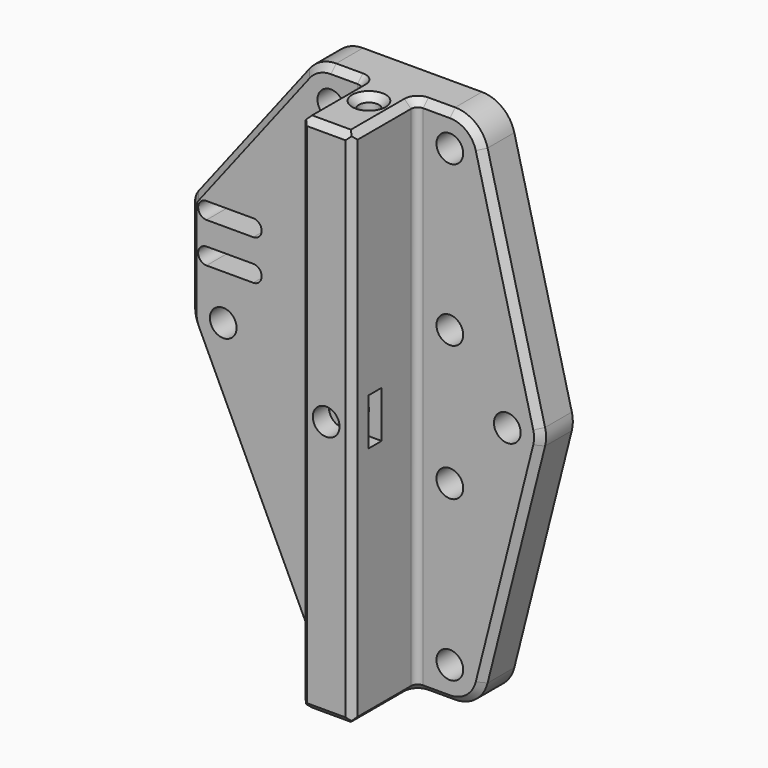
from build123d import *

# Parameters (mm, degrees)
F0_R          = 2
F1_DEPTH      = 6
F2_W          = 7.8
F2_H          = 78
F3_DEPTH      = 12
F4_R          = 2
F5_DEPTH      = 12
F6_W          = 2.5
F6_H          = 7
F7_DEPTH      = 33.901
F8_R          = 1.5
F9_DEPTH      = 39.001
F9_DEPTH_BACK = 39.001
F10_DEPTH     = 2.5
F11_SIZE      = 1
F12_R         = 1
F13_SIZE      = 1
F14_SIZE      = 1
F15_W         = 13.75
F15_H         = 4
F16_DEPTH     = 2


# Not quite as in the source:
# - a feature names something its author has since deleted; it is built from what else it names


with BuildPart() as f1:
    # F0 (on Front) → F1 (new body)
    with BuildSketch(Plane.XZ):
        with BuildLine():
            Line((22.3473393815, 1.2260917259), (13.7473393815, 35.2260917259))
            ThreePointArc((13.7473393815, 35.2260917259), (11.9716071828, 37.9452793709), (8.9, 39))
            Line((8.9, 39), (-8.9, 39))
            ThreePointArc((-8.9, 39), (-11.1047505583, 38.4876580725), (-12.8576666563, 37.0556299903))
            Line((-12.8576666563, 37.0556299903), (-29.4788333281, 15.5278149952))
            ThreePointArc((-29.4788333281, 15.5278149952), (-29.8661237626, 14.8071296921), (-30, 14))
            Line((-30, 14), (-30, 0))
            ThreePointArc((-30, 0), (-29.8782578321, -1.0966314436), (-29.5189597908, -2.1398603715))
            Line((-29.5189597908, -2.1398603715), (-13.4189597908, -36.1398603715))
            ThreePointArc((-13.4189597908, -36.1398603715), (-11.5740136632, -38.2248847237), (-8.9, -39))
            Line((-8.9, -39), (8.9, -39))
            ThreePointArc((8.9, -39), (11.9716071828, -37.9452793709), (13.7473393815, -35.2260917259))
            Line((13.7473393815, -35.2260917259), (22.3473393815, -1.2260917259))
            ThreePointArc((22.3473393815, -1.2260917259), (22.5, 0), (22.3473393815, 1.2260917259))
        make_face()
        with Locations((-8.9, -34)):
            Circle(F0_R, mode=Mode.SUBTRACT)
        with Locations((-8.9, -10.1)):
            Circle(F0_R, mode=Mode.SUBTRACT)
        with Locations((8.9, -34)):
            Circle(F0_R, mode=Mode.SUBTRACT)
        with Locations((8.9, -10.1)):
            Circle(F0_R, mode=Mode.SUBTRACT)
        with Locations((-25, 0)):
            Circle(F0_R, mode=Mode.SUBTRACT)
        with BuildLine():
            ThreePointArc((-20.5, 9.25), (-19.25, 8), (-20.5, 6.75))
            Line((-20.5, 6.75), (-27.5, 6.75))
            ThreePointArc((-27.5, 6.75), (-28.75, 8), (-27.5, 9.25))
            Line((-27.5, 9.25), (-20.5, 9.25))
        make_face(mode=Mode.SUBTRACT)
        with BuildLine():
            ThreePointArc((-27.5, 12.75), (-28.75, 14), (-27.5, 15.25))
            Line((-27.5, 15.25), (-20.5, 15.25))
            ThreePointArc((-20.5, 15.25), (-19.25, 14), (-20.5, 12.75))
            Line((-20.5, 12.75), (-27.5, 12.75))
        make_face(mode=Mode.SUBTRACT)
        with Locations((-8.9, 10.1)):
            Circle(F0_R, mode=Mode.SUBTRACT)
        with Locations((-8.9, 34)):
            Circle(F0_R, mode=Mode.SUBTRACT)
        with Locations((8.9, 10.1)):
            Circle(F0_R, mode=Mode.SUBTRACT)
        with Locations((17.5, 0)):
            Circle(F0_R, mode=Mode.SUBTRACT)
        with Locations((8.9, 34)):
            Circle(F0_R, mode=Mode.SUBTRACT)
    extrude(amount=F1_DEPTH)

    # F2 (on face) → F3 (join)
    with BuildSketch(Plane.XZ.offset(6)):
        Rectangle(F2_W, F2_H)
    extrude(amount=F3_DEPTH)

    # F4 (on face) → F5 (cut, through all)
    with BuildSketch(Plane.XZ.offset(18)):
        Circle(F4_R)
    extrude(amount=-F5_DEPTH, mode=Mode.SUBTRACT)

    # F6 (on face) → F7 (cut, through all)
    with BuildSketch(Plane.YZ.offset(3.9)):
        with Locations((-13.75, 0)):
            Rectangle(F6_W, F6_H)
    extrude(amount=-F7_DEPTH, mode=Mode.SUBTRACT)

    # F8 (on Top) → F9 (cut, two sides)
    with BuildSketch(Plane.XY) as f9_sk:
        with Locations((0, -10)):
            Circle(F8_R)
    extrude(amount=-F9_DEPTH, mode=Mode.SUBTRACT)
    extrude(f9_sk.sketch, amount=F9_DEPTH_BACK, mode=Mode.SUBTRACT)

    # F10 (add): a face of the model
    f10_faces = [f1.faces().sort_by_distance(p)[0] for p in [
        (0, -6, 0),
    ]]
    extrude(f10_faces, amount=F10_DEPTH)

    # F11
    f11_edges = [f1.edges().sort_by_distance(p)[0] for p in [
        (3.9, -18, 0),
        (-3.9, -18, 0),
    ]]
    chamfer(f11_edges, length=F11_SIZE)

    # F12
    f12_edges = [f1.edges().sort_by_distance(p)[0] for p in [
        (-3.9, -6, 0),
        (3.9, -6, 0),
    ]]
    fillet(f12_edges, radius=F12_R)

    # F13 (call 1 of 4: OpenCascade refuses the feature's edges together)
    f13_edges = [f1.edges().sort_by_distance(p)[0] for p in [
        (18.047339, -6, 18.226092),
    ]]
    chamfer(f13_edges, length=F13_SIZE)

    # F13#2 (call 2 of 4)
    f13_2_edges = [f1.edges().sort_by_distance(p)[0] for p in [
        (0, -18, -39),
    ]]
    chamfer(f13_2_edges, length=F13_SIZE)

    # F13#3 (call 3 of 4)
    f13_3_edges = [f1.edges().sort_by_distance(p)[0] for p in [
        (0, -18, 39),
    ]]
    chamfer(f13_3_edges, length=F13_SIZE)

    # F13#4 (call 4 of 4)
    f13_4_edges = [f1.edges().sort_by_distance(p)[0] for p in [
        (-30, -6, 7),
    ]]
    chamfer(f13_4_edges, length=F13_SIZE)

    # F14
    f14_edges = [f1.edges().sort_by_distance(p)[0] for p in [
        (-1.5, -10, 39),
    ]]
    chamfer(f14_edges, length=F14_SIZE)

    # F15 (on face) → F16 (cut)
    with BuildSketch(Plane(origin=(0, 0, 0), x_dir=(-1, 0, 0), z_dir=(0, 1, 0))):
        with BuildLine():
            Line((29.1142693598, 16), (16.25, 16))
            Line((16.25, 16), (16.25, 12))
            Line((16.25, 12), (30, 12))
            Line((30, 12), (30, 14))
            ThreePointArc((30, 14), (29.8661237626, 14.8071296921), (29.4788333281, 15.5278149952))
            Line((29.4788333281, 15.5278149952), (29.1142693598, 16))
        make_face()
        with BuildLine():
            Line((20.5, 15.25), (27.5, 15.25))
            ThreePointArc((27.5, 15.25), (28.75, 14), (27.5, 12.75))
            Line((27.5, 12.75), (20.5, 12.75))
            ThreePointArc((20.5, 12.75), (19.25, 14), (20.5, 15.25))
        make_face(mode=Mode.SUBTRACT)
        with Locations((23.125, 8)):
            Rectangle(F15_W, F15_H)
        with BuildLine():
            Line((27.5, 6.75), (20.5, 6.75))
            ThreePointArc((20.5, 6.75), (19.25, 8), (20.5, 9.25))
            Line((20.5, 9.25), (27.5, 9.25))
            ThreePointArc((27.5, 9.25), (28.75, 8), (27.5, 6.75))
        make_face(mode=Mode.SUBTRACT)
    extrude(amount=-F16_DEPTH, mode=Mode.SUBTRACT)


solid = f1.part
